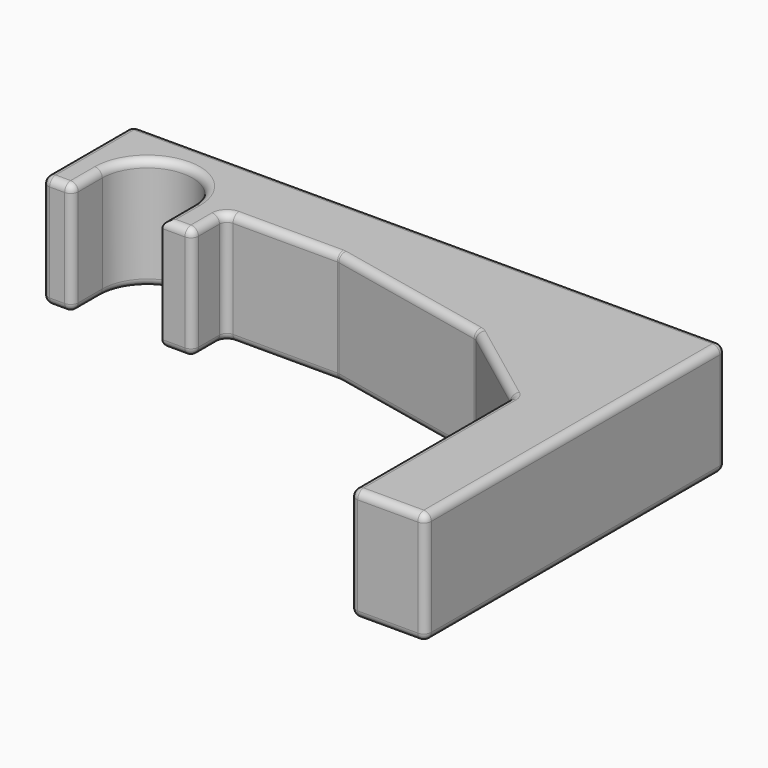
from build123d import *

# Parameters (mm, degrees)
F1_DEPTH = 30
F2_W     = 20.25
F2_H     = 20.25
F3_DEPTH = 15
F4_R     = 2


# Not quite as in the source:
# - a feature names something its author has since deleted; it is built from what else it names


with BuildPart() as f1:
    # F0 (on Top) → F1 (new body)
    with BuildSketch(Plane.XY):
        Polygon((-12, -5), (-12, 5), (-12, 25), (-20, 25), (-20, -5), align=None)
        with BuildLine():
            ThreePointArc((-12, 5), (0, 17), (12, 5))
            Line((12, 5), (12, 25))
            Line((12, 25), (-12, 25))
            Line((-12, 25), (-12, 5))
        make_face()
        Polygon((12, 25), (12, 5), (12, -5), (20, -5), (20, 6), (50, 6), (94.016642033, -3.3560260868), (118, -21.3781941203), (118, -75), (138, -75), (138, -15), (138, 25), align=None)
    extrude(amount=F1_DEPTH)

    # F2 (on face) → F3 (cut)
    with BuildSketch(Plane(origin=(118, 0, 0), x_dir=(0, -1, 0), z_dir=(-1, 0, 0))):
        with Locations((60, 15)):
            Rectangle(F2_W, F2_H)
    extrude(amount=-F3_DEPTH, mode=Mode.SUBTRACT)

    # F4
    f4_edges = [f1.edges().sort_by_distance(p)[0] for p in [
        (20, -5, 15),
        (20, 6, 15),
        (20, 0.5, 0),
        (20, 0.5, 30),
        (50, 6, 15),
        (35, 6, 0),
        (35, 6, 30),
        (94.016642, -3.356026, 15),
        (118, -21.378194, 15),
        (106.008321, -12.36711, 0),
        (106.008321, -12.36711, 30),
        (118, -48.189097, 0),
        (118, -48.189097, 30),
        (118, -75, 15),
        (118, -60, 4.875),
        (118, -49.875, 15),
        (118, -60, 25.125),
        (118, -70.125, 15),
        (138, -75, 15),
        (128, -75, 0),
        (128, -75, 30),
        (-20, 10, 30),
        (-16, -5, 30),
        (-12, 0, 30),
        (0, 17, 30),
        (12, 0, 30),
        (16, -5, 30),
        (72.008321, 1.321987, 30),
        (138, -25, 30),
        (59, 25, 30),
        (-20, 10, 0),
        (-16, -5, 0),
        (-12, 0, 0),
        (0, 17, 0),
        (12, 0, 0),
        (16, -5, 0),
        (72.008321, 1.321987, 0),
        (138, -25, 0),
        (59, 25, 0),
        (-20, -5, 15),
        (-12, -5, 15),
        (138, 25, 15),
        (-20, 25, 15),
    ]]
    fillet(f4_edges, radius=F4_R)


solid = f1.part
